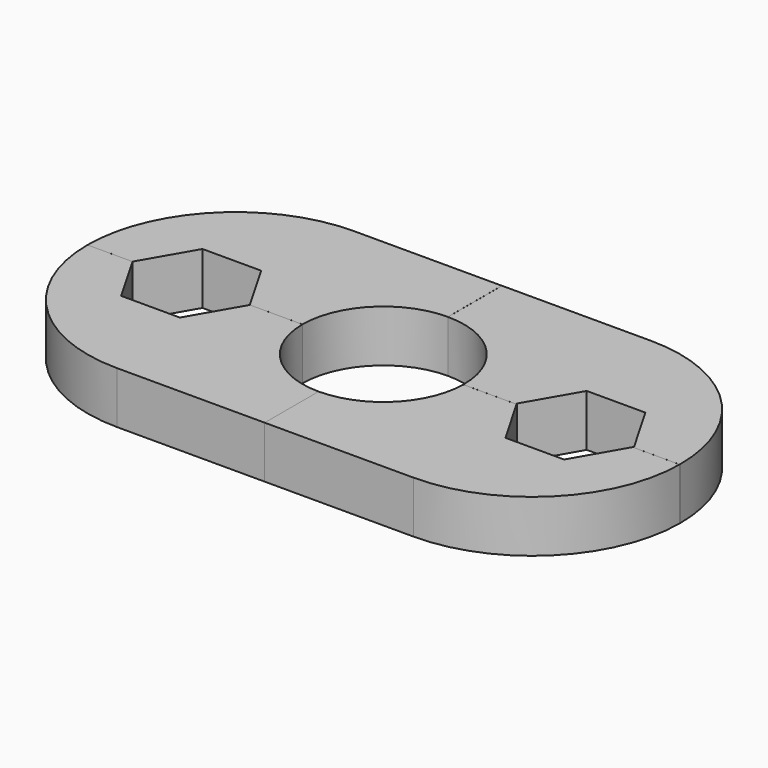
from build123d import *

# Parameters (mm, degrees)
F1_DEPTH      = 7
F2_T1_DEPTH   = 107
F2_2_T1_DEPTH = 107
F2_3_T1_DEPTH = 107
F2_4_T1_DEPTH = 107


# Not quite as in the source:
# - a fillet or chamfer that OpenCascade refuses, or shapes differently, is made with other operations: its cross-section is extruded or revolved along the edge and cut away or added


with BuildPart() as f1:
    # F0 (on Top) → F1 (new body)
    with BuildSketch(Plane.XY):
        with BuildLine():
            Line((-0.0071190066, 20.0072696805), (-0.0071190066, 20))
            Line((-0.0071190066, 20), (0, 20))
            Line((0, 20), (0, 10.9))
            ThreePointArc((0, 10.9), (7.7074639149, 7.7074639149), (10.9, 0))
            ThreePointArc((10.9, 0), (10.899781335, -0.0690423694), (10.8991253488, -0.1380819688))
            Line((10.8991253488, -0.1380819688), (18.0797216618, -0.1380819688))
            Line((18.0797216618, -0.1380819688), (18, 0))
            Line((18, 0), (21.9548493439, 6.85))
            Line((21.9548493439, 6.85), (29.8645480318, 6.85))
            Line((29.8645480318, 6.85), (33.8193973758, 0))
            Line((33.8193973758, 0), (33.739675714, -0.1380819688))
            Line((33.739675714, -0.1380819688), (40.0763135217, -0.1380819688))
            Line((40.0763135217, -0.1380819688), (40.0763135217, 20.0072696805))
            Line((40.0763135217, 20.0072696805), (-0.0071190066, 20.0072696805))
        make_face()
    extrude(amount=F1_DEPTH)

    # F2#4: fillet of radius 20 on 1 edges, made by hand

    # F2_4_s2 → F2_4_t1 (cut)
    with BuildSketch(Plane.XY.offset(-50)):
        with BuildLine():
            ThreePointArc((20.0763135217, 20.0072696805), (34.2184491454, 14.1494053042), (40.0763135217, 0.0072696805))
            Line((40.0763135217, 0.0072696805), (40.0763135217, 20.0072696805))
            Line((40.0763135217, 20.0072696805), (20.0763135217, 20.0072696805))
        make_face()
    extrude(amount=F2_4_T1_DEPTH, mode=Mode.SUBTRACT)


with BuildPart() as f1b:
    # F0 (on Top) → F1, piece 2 (new body)
    with BuildSketch(Plane.XY):
        with BuildLine():
            Line((-39.8988322914, 0), (-33.8193973758, 0))
            Line((-33.8193973758, 0), (-29.8645480318, 6.85))
            Line((-29.8645480318, 6.85), (-21.9548493439, 6.85))
            Line((-21.9548493439, 6.85), (-18, 0))
            Line((-18, 0), (-10.9, 0))
            ThreePointArc((-10.9, 0), (-7.709980453, 7.7049465549), (-0.0071190066, 10.8999976752))
            Line((-0.0071190066, 10.8999976752), (-0.0071190066, 20))
            Line((-0.0071190066, 20), (-39.8988322914, 20))
            Line((-39.8988322914, 20), (-39.8988322914, 0))
        make_face()
    extrude(amount=F1_DEPTH)

    # F2: fillet of radius 20 on 1 edges, made by hand

    # F2_s2 → F2_t1 (cut)
    with BuildSketch(Plane.XY.offset(-50)):
        with BuildLine():
            ThreePointArc((-19.8988322914, 20), (-34.0409679151, 14.1421356237), (-39.8988322914, 0))
            Line((-39.8988322914, 0), (-39.8988322914, 20))
            Line((-39.8988322914, 20), (-19.8988322914, 20))
        make_face()
    extrude(amount=F2_T1_DEPTH, mode=Mode.SUBTRACT)


with BuildPart() as f1c:
    # F0 (on Top) → F1, piece 3 (new body)
    with BuildSketch(Plane.XY):
        with BuildLine():
            Line((-29.8645480318, -6.85), (-33.8183725607, -0.0017750319))
            Line((-33.8183725607, -0.0017750319), (-39.897811533, -0.0017750319))
            Line((-39.897811533, -0.0017750319), (-39.897811533, -19.9902126039))
            Line((-39.897811533, -19.9902126039), (-0.0018734138, -19.9902126039))
            Line((-0.0018734138, -19.9902126039), (-0.0018734138, -10.899999839))
            ThreePointArc((-0.0018734138, -10.899999839), (-7.7074986981, -7.7074291316), (-10.8999998555, -0.0017750319))
            Line((-10.8999998555, -0.0017750319), (-18.0010248151, -0.0017750319))
            Line((-18.0010248151, -0.0017750319), (-21.9548493439, -6.85))
            Line((-21.9548493439, -6.85), (-29.8645480318, -6.85))
        make_face()
    extrude(amount=F1_DEPTH)

    # F2#2: fillet of radius 20 on 1 edges, made by hand

    # F2_2_s2 → F2_2_t1 (cut)
    with BuildSketch(Plane.XY.offset(-50)):
        with BuildLine():
            ThreePointArc((-39.897811533, 0.0097873961), (-34.0399471567, -14.1323482276), (-19.897811533, -19.9902126039))
            Line((-19.897811533, -19.9902126039), (-39.897811533, -19.9902126039))
            Line((-39.897811533, -19.9902126039), (-39.897811533, 0.0097873961))
        make_face()
    extrude(amount=F2_2_T1_DEPTH, mode=Mode.SUBTRACT)


with BuildPart() as f1d:
    # F0 (on Top) → F1, piece 4 (new body)
    with BuildSketch(Plane.XY):
        with BuildLine():
            ThreePointArc((10.8990613818, -0.1430419341), (7.6563698297, -7.7582215121), (-0.0009950386, -10.8999999546))
            Line((-0.0009950386, -10.8999999546), (-0.0009950386, -19.9906610558))
            Line((-0.0009950386, -19.9906610558), (40.0799419763, -19.9906610558))
            Line((40.0799419763, -19.9906610558), (40.0799419763, -0.1380819688))
            Line((40.0799419763, -0.1380819688), (40.0763135217, -0.1380819688))
            Line((40.0763135217, -0.1380819688), (40.0763135217, -0.1430419341))
            Line((40.0763135217, -0.1430419341), (33.7368120767, -0.1430419341))
            Line((33.7368120767, -0.1430419341), (29.8645480318, -6.85))
            Line((29.8645480318, -6.85), (21.9548493439, -6.85))
            Line((21.9548493439, -6.85), (18.0825852991, -0.1430419341))
            Line((18.0825852991, -0.1430419341), (10.8990613818, -0.1430419341))
        make_face()
    extrude(amount=F1_DEPTH)

    # F2#3: fillet of radius 20 on 1 edges, made by hand

    # F2_3_s2 → F2_3_t1 (cut)
    with BuildSketch(Plane.XY.offset(-50)):
        with BuildLine():
            ThreePointArc((20.0799419763, -19.9906610558), (34.2220776, -14.1327966795), (40.0799419763, 0.0093389442))
            Line((40.0799419763, 0.0093389442), (40.0799419763, -19.9906610558))
            Line((40.0799419763, -19.9906610558), (20.0799419763, -19.9906610558))
        make_face()
    extrude(amount=F2_3_T1_DEPTH, mode=Mode.SUBTRACT)


solid = Compound([f1.part, f1b.part, f1c.part, f1d.part])
